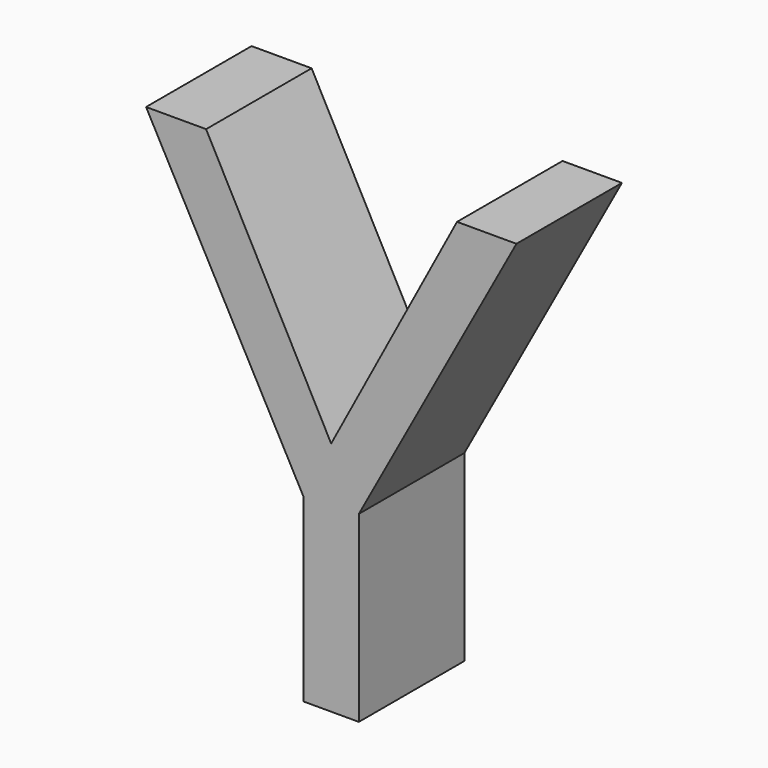
from build123d import *

# Parameters (mm, degrees)
F0_TEXT_SIZE = 50.1554097152
F1_DEPTH     = 10


# Not quite as in the source:
# - Text() gives the source's letters only with a copy of the font that has no kerning and outlines rounded to 1/6400 em; it was checked with that copy


with BuildPart() as f1:
    # F0 (on Front) → F1 (new body)
    with BuildSketch(Plane.XZ):
        with Locations((-31.3392942893, 0)):
            Text('Y', F0_TEXT_SIZE, font='Open Sans', text_align=(TextAlign.LEFT, TextAlign.BOTTOM))
    extrude(amount=F1_DEPTH)


solid = f1.part
